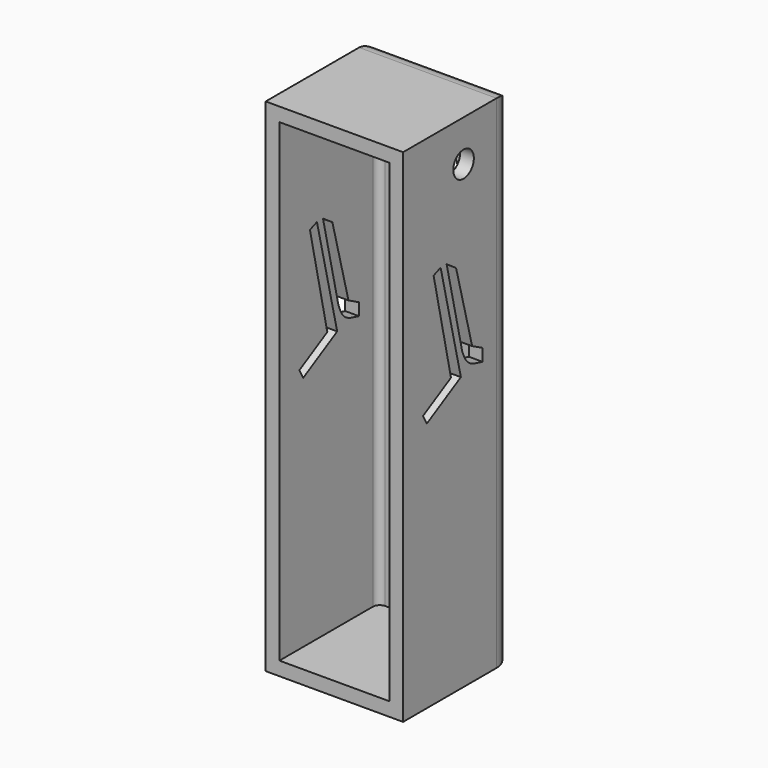
from build123d import *

# Parameters (mm, degrees)
F0_W     = 25.4
F0_H     = 92.71
F1_DEPTH = 25.4
F2_R     = 3.81
F3_T     = -2.54
F4_R     = 2.3749
F5_DEPTH = 33.89182
F7_DEPTH = 25.4
F9_DEPTH = 41.87188


# Not quite as in the source:
# - a feature names something its author has since deleted; it is built from what else it names


with BuildPart() as f1:
    # F0 (on Front) → F1 (new body)
    with BuildSketch(Plane.XZ):
        with Locations((-41.9686666963, 12.4836304921)):
            Rectangle(F0_W, F0_H)
    extrude(amount=F1_DEPTH)

    # F2
    f2_edges = [f1.edges().sort_by_distance(p)[0] for p in [
        (-41.968667, 0, 58.83863),
        (-29.268667, 0, 12.48363),
        (-54.668667, 0, 12.48363),
    ]]
    fillet(f2_edges, radius=F2_R)

    # F3
    f3_openings = [f1.faces().sort_by_distance(p)[0] for p in [
        (-41.968667, -25.4, 12.48363),
    ]]
    offset(amount=F3_T, openings=f3_openings)

    # F4 (on face) → F5 (cut)
    with BuildSketch(Plane.YZ.offset(-29.2686666963)):
        with Locations((-11.43, 51.2186304921)):
            Circle(F4_R)
    extrude(amount=-F5_DEPTH, mode=Mode.SUBTRACT)

    # F6 (on face) → F7 (cut)
    with BuildSketch(Plane(origin=(0, 0, 0), x_dir=(-1, 0, 0), z_dir=(0, 1, 0))):
        with BuildLine():
            Line((44.6058399975, 26.3032466173), (38.2379107177, 26.3032466173))
            Line((38.2379107177, 26.3032466173), (37.1410762263, 24.0397093349))
            add(Edge.make_bspline(
                [(37.1410762263, 24.0397093349), (37.339065454, 24.3792086296), (38.2035071777, 25.5814413695), (40.3849287439, 26.669887034), (42.7800860183, 26.0425383856), (44.011480676, 25.9258376474)],
                knots=[0.8982713577, 0.8982713577, 0.8982713577, 0.8982713577, 0.9129794329, 0.9539867719, 1, 1, 1, 1], degree=3))
            Line((44.011480676, 25.9258376474), (44.6058399975, 24.8313006014))
            Line((44.6058399975, 24.8313006014), (44.6058399975, 26.3032466173))
        make_face()
        with BuildLine():
            add(Edge.make_bspline(
                [(42.7850283084, 18.2644031587), (41.6281881248, 17.7122917547), (39.3421934753, 18.0628655754), (36.5998069985, 19.4455682818), (36.1790606743, 21.3684728246), (36.540582062, 22.7181603941), (36.7136490494, 23.1576278923)],
                knots=[0.7466786433, 0.7466786433, 0.7466786433, 0.7466786433, 0.7915745353, 0.8322226711, 0.8681939908, 0.8860298615, 0.8860298615, 0.8860298615, 0.8860298615], degree=3))
            Line((36.7136490494, 23.1576278923), (35.1822041317, 19.9971850961))
            Line((35.1822041317, 19.9971850961), (38.4076647026, 16.2012871028))
            add(Edge.make_bspline(
                [(38.4076647026, 16.2012871028), (38.3331463783, 16.3354515994), (38.1281105022, 16.8597586898), (38.0130316953, 18.2731129731), (40.1443547311, 17.9923088512), (40.2538308709, 15.6035026602), (43.1039682699, 16.2758181544), (45.8152821105, 17.1489055351), (45.7320952633, 20.6477240715), (44.1444598015, 19.0789790813), (43.2506561167, 18.5227281558)],
                knots=[0.4950053944, 0.4950053944, 0.4950053944, 0.4950053944, 0.505624299, 0.5328808409, 0.5614669556, 0.5935350141, 0.6306867364, 0.6713872521, 0.705194827, 0.7406037078, 0.7406037078, 0.7406037078, 0.7406037078], degree=3))
            add(Edge.make_bspline(
                [(43.2506561167, 18.5227281558), (43.0973104129, 18.4272947949), (42.9415622179, 18.3391102426), (42.7850283084, 18.2644031587)],
                knots=[0.7406037078, 0.7406037078, 0.7406037078, 0.7406037078, 0.7466786433, 0.7466786433, 0.7466786433, 0.7466786433], degree=3))
        make_face()
        with BuildLine():
            Line((48.8165095448, 19.9971850961), (45.9266088615, 25.2345095571))
            Line((45.9266088615, 25.2345095571), (45.9266088615, 23.5216511982))
            Line((45.9266088615, 23.5216511982), (43.2445396799, 23.5216511982))
            add(Edge.make_bspline(
                [(43.2445396799, 23.5216511982), (42.7081827873, 23.8075607265), (42.1988237282, 23.6134021644), (41.3260156155, 23.9456441334), (38.606688661, 22.6279980556), (38.8696183743, 21.2171215213), (38.9977403957, 20.4411421944), (41.0886389354, 19.0960129486), (43.9500070475, 21.2758052217), (45.9447358431, 23.2877508917), (48.9073126692, 21.0534189), (47.1000899952, 18.4437720499), (45.9026933546, 16.7229533606), (42.6849572511, 14.5068511007), (40.7344690342, 14.5241406274), (39.3098813456, 15.2865012258), (38.8615001809, 15.667188749)],
                knots=[0, 0, 0, 0, 0.0251384715, 0.0472797991, 0.0868576025, 0.1130533046, 0.1338423204, 0.1676504586, 0.212200273, 0.2507501602, 0.2893385494, 0.3281494521, 0.3649907492, 0.4113089163, 0.444795994, 0.4795115688, 0.4795115688, 0.4795115688, 0.4795115688], degree=3))
            Line((38.8615001809, 15.667188749), (41.7874008417, 12.223829203))
            Line((41.7874008417, 12.223829203), (48.8165095448, 19.9971850961))
        make_face()
        with BuildLine():
            Line((38.6650130318, 3.0435510572), (34.0940020009, 3.0435510572))
            add(Edge.make_bspline(
                [(34.0940020009, 3.0435510572), (35.3064836638, 2.0585014096), (36.6486475232, 1.0417361836), (37.0877473703, 0.4615400411)],
                knots=[0, 0, 0, 0, 0.6725136257, 0.6725136257, 0.6725136257, 0.6725136257], degree=3))
            add(Edge.make_bspline(
                [(37.0877473703, 0.4615400411), (37.2488894729, 0.2486180213), (37.2884101705, 0.0944915516), (37.3894860772, -0.1281914716)],
                knots=[0.6725136257, 0.6725136257, 0.6725136257, 0.6725136257, 0.9193145762, 0.9193145762, 0.9193145762, 0.9193145762], degree=3))
            Line((37.3894860772, -0.1281914716), (37.5147564062, -0.3730253592))
            Line((37.5147564062, -0.3730253592), (39.4241169946, -0.3710518407))
            add(Edge.make_bspline(
                [(39.4241169946, -0.3710518407), (40.2193717367, -0.172634483), (41.7498927591, 0.9430647342), (41.9405885041, -4.0000835434), (41.9386439387, -2.1187349198)],
                knots=[0.343503575, 0.343503575, 0.343503575, 0.343503575, 0.7050061608, 1, 1, 1, 1], degree=3))
            add(Edge.make_bspline(
                [(41.9386439387, -2.1187349198), (41.9405885041, -4.0000835434), (42.1065657162, 0.9442821093), (44.5176392833, -0.7547523857), (45.7934533434, -0.3571810129), (46.3589132856, -0.3638840226)],
                knots=[0, 0, 0, 0, 0.2949938392, 0.656496425, 1, 1, 1, 1], degree=3))
            add(Edge.make_bspline(
                [(46.3589132856, -0.3638840226), (46.5070234145, -0.0989215722), (46.6363921506, 0.6669917593), (48.5601159674, 2.0747068345), (49.7725976303, 3.0597564821)],
                knots=[0, 0, 0, 0, 0.3274863743, 1, 1, 1, 1], degree=3))
            Line((49.7725976303, 3.0597564821), (45.201596366, 3.0503072816))
            add(Edge.make_bspline(
                [(45.201596366, 3.0503072816), (45.0298966378, 2.799615514), (44.8833484647, 2.1805451993), (43.5805476832, 1.9102075859), (42.4006120518, 2.0733394322), (42.5828706814, 3.1590564965), (42.6892745175, 3.7842430815)],
                knots=[0, 0, 0, 0, 0.2185913056, 0.4809582477, 0.7068513006, 1, 1, 1, 1], degree=3))
            add(Edge.make_bspline(
                [(41.1758123193, 3.7826787643), (41.2675346128, 3.4547941063), (41.522874003, 3.0072416083), (41.9331378394, 3.1648265114), (42.3440419659, 3.0080384673), (42.597552224, 3.4563584235), (42.6892745175, 3.7842430815)],
                knots=[0, 0, 0, 0, 0.3003096746, 0.5, 0.6996903254, 1, 1, 1, 1], degree=3))
            add(Edge.make_bspline(
                [(41.1758123193, 3.7826787643), (41.2822161554, 3.1574921793), (41.468490602, 2.0724705891), (40.2882148417, 1.906733948), (38.9853825849, 2.1746547143), (38.83671276, 2.7928592896), (38.6650130318, 3.0435510572)],
                knots=[0, 0, 0, 0, 0.2931486994, 0.5190417523, 0.7814086944, 1, 1, 1, 1], degree=3))
        make_face()
        with BuildLine():
            add(Edge.make_bspline(
                [(37.0877473703, 0.4615400411), (37.2488894729, 0.2486180213), (37.2884101705, 0.0944915516), (37.3894860772, -0.1281914716)],
                knots=[0.6725136257, 0.6725136257, 0.6725136257, 0.6725136257, 0.9193145762, 0.9193145762, 0.9193145762, 0.9193145762], degree=3))
            Line((37.0877473703, 0.4615400411), (37.3894860772, -0.1281914716))
        make_face()
        with BuildLine():
            Line((41.9686666963, 48.4663217602), (41.9686666963, 49.8393438756))
            Line((41.9686666963, 49.8393438756), (37.418499589, 49.8393438756))
            Line((37.418499589, 49.8393438756), (37.418499589, 47.1883751452))
            Line((37.418499589, 47.1883751452), (38.8069276568, 47.1883751452))
            ThreePointArc((38.8069276568, 47.1883751452), (40.2635463703, 48.1347545839), (41.9686666963, 48.4663217602))
        make_face()
        with BuildLine():
            Line((46.5188338037, 49.8393438756), (41.9686666963, 49.8393438756))
            Line((41.9686666963, 49.8393438756), (41.9686666963, 48.4663217602))
            ThreePointArc((41.9686666963, 48.4663217602), (43.6737870223, 48.1347545839), (45.1304057359, 47.1883751452))
            Line((45.1304057359, 47.1883751452), (46.5188338037, 47.1883751452))
            Line((46.5188338037, 47.1883751452), (46.5188338037, 49.8393438756))
        make_face()
        with BuildLine():
            Line((41.9686666963, 39.3659875455), (41.9686666963, 48.4663217602))
            ThreePointArc((41.9686666963, 48.4663217602), (40.2635463703, 48.1347545839), (38.8069276568, 47.1883751452))
            ThreePointArc((38.8069276568, 47.1883751452), (37.4206220872, 44.0551184562), (38.6130492157, 40.8430695534))
            ThreePointArc((38.6130492157, 40.8430695534), (40.135504133, 39.751597567), (41.9686666963, 39.3659875455))
        make_face()
        with BuildLine():
            ThreePointArc((45.1304057359, 47.1883751452), (43.6737870223, 48.1347545839), (41.9686666963, 48.4663217602))
            Line((41.9686666963, 48.4663217602), (41.9686666963, 39.3659875455))
            ThreePointArc((41.9686666963, 39.3659875455), (43.8018292596, 39.751597567), (45.3242841769, 40.8430695534))
            ThreePointArc((45.3242841769, 40.8430695534), (46.2096949319, 42.2676097763), (46.5188338037, 43.9161546528))
            ThreePointArc((46.5188338037, 43.9161546528), (46.15736946, 45.6934531259), (45.1304057359, 47.1883751452))
        make_face()
        with BuildLine():
            Line((41.9686666963, 38.4213812649), (41.9686666963, 39.3659875455))
            ThreePointArc((41.9686666963, 39.3659875455), (40.135504133, 39.751597567), (38.6130492157, 40.8430695534))
            Line((38.6130492157, 40.8430695534), (37.418499589, 40.8430695534))
            Line((37.418499589, 40.8430695534), (37.418499589, 38.4213812649))
            Line((37.418499589, 38.4213812649), (41.9686666963, 38.4213812649))
        make_face()
        with BuildLine():
            ThreePointArc((45.3242841769, 40.8430695534), (43.8018292596, 39.751597567), (41.9686666963, 39.3659875455))
            Line((41.9686666963, 39.3659875455), (41.9686666963, 38.4213812649))
            Line((41.9686666963, 38.4213812649), (46.5188338037, 38.4213812649))
            Line((46.5188338037, 38.4213812649), (46.5188338037, 40.8430695534))
            Line((46.5188338037, 40.8430695534), (45.3242841769, 40.8430695534))
        make_face()
    extrude(amount=-F7_DEPTH, mode=Mode.SUBTRACT)

    # F8 (on face) → F9 (cut)
    with BuildSketch(Plane(origin=(-54.6686666963, 0, 0), x_dir=(0, -1, 0), z_dir=(-1, 0, 0))):
        with BuildLine():
            Line((11.7656327784, 20.9736730903), (15.33928141, 36.5336947143))
            Line((15.33928141, 36.5336947143), (13.1652783602, 35.0378602743))
            Line((13.1652783602, 35.0378602743), (9.4449697062, 20.794250071))
            add(Edge.make_bspline(
                [(7.0266528055, 19.5226483047), (7.8327584391, 19.9465155602), (8.6388640727, 20.3703828156), (9.4449697062, 20.794250071)],
                knots=[0, 0, 0, 0, 2.7322568848, 2.7322568848, 2.7322568848, 2.7322568848], degree=3))
            Line((7.0266528055, 19.5226483047), (7.0266528055, 17.2587186098))
            add(Edge.make_bspline(
                [(11.7656327784, 20.9736730903), (11.4196888419, 20.0493595473), (10.6857841803, 18.0884695114), (8.2920446058, 17.5456610231), (7.0266528055, 17.2587186098)],
                knots=[0, 0, 0, 0, 0.4713744913, 1, 1, 1, 1], degree=3))
        make_face()
        Polygon((18.3508805931, 35.8983948827), (16.7308822274, 36.5336947143), (12.0496712625, 16.8081112206), (19.9097655714, 12.4404029921), (20.8017168623, 14.0455517105), (14.3370925642, 17.6378232064), align=None)
    extrude(amount=-F9_DEPTH, mode=Mode.SUBTRACT)


solid = f1.part
